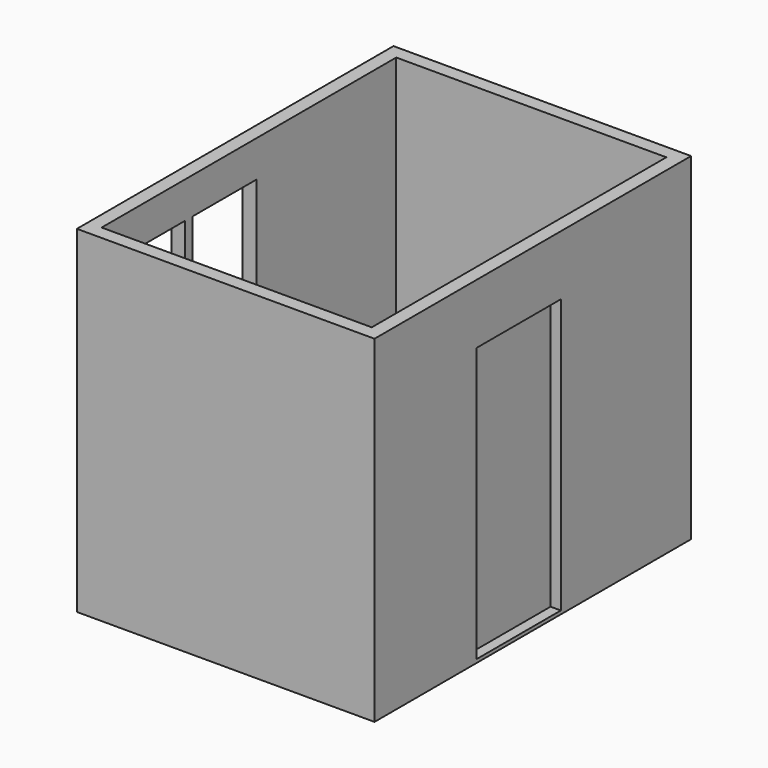
from build123d import *

# Parameters (mm, degrees)
F0_W     = 100
F0_H     = 580
F0_H_2   = 68
F0_H_3   = 765
F1_DEPTH = 2430
F2_W     = 580
F2_H     = 890
F3_DEPTH = 100.001
F4_W     = 765
F4_H     = 1994
F5_DEPTH = 100
F6_W     = 760
F6_H     = 1989
F7_DEPTH = 25
F8_DEPTH = 25


with BuildPart() as f1:
    # F0 (on Top) → F1 (new body)
    with BuildSketch(Plane.XY):
        Polygon((0, -2680), (-1966, -2680), (-1966, -2500), (-2066, -2500), (-2066, -2780), (100, -2780), (100, -1850), (0, -1850), align=None)
        with Locations((-2016, -2210)):
            Rectangle(F0_W, F0_H)
        with Locations((-2016, -1886)):
            Rectangle(F0_W, F0_H_2)
        with Locations((-2016, -1562)):
            Rectangle(F0_W, F0_H)
        with Locations((50, -1467.5)):
            Rectangle(F0_W, F0_H_3)
        Polygon((0, 0), (0, -1085), (100, -1085), (100, 100), (-2066, 100), (-2066, -1272), (-1966, -1272), (-1966, 0), align=None)
    extrude(amount=F1_DEPTH)

    # F2 (on face) → F3 (cut, through all)
    with BuildSketch(Plane.YZ.offset(-1966)):
        with Locations((-1562, 1720)):
            Rectangle(F2_W, F2_H)
        with Locations((-2210, 1720)):
            Rectangle(F2_W, F2_H)
    extrude(amount=-F3_DEPTH, mode=Mode.SUBTRACT)

    # F4 (on face) → F5 (cut, through all)
    with BuildSketch(Plane.YZ.offset(100)):
        with Locations((-1467.5, 997)):
            Rectangle(F4_W, F4_H)
    extrude(amount=-F5_DEPTH, mode=Mode.SUBTRACT)

    # F0 (on Top) → F8 (join)
    with BuildSketch(Plane.XY):
        Polygon((0, -2680), (-1966, -2680), (-1966, -2500), (-2066, -2500), (-2066, -2780), (100, -2780), (100, -1850), (0, -1850), align=None)
        with Locations((-2016, -2210)):
            Rectangle(F0_W, F0_H)
        with Locations((50, -1467.5)):
            Rectangle(F0_W, F0_H_3)
        with Locations((-2016, -1886)):
            Rectangle(F0_W, F0_H_2)
        Polygon((0, 0), (0, -1085), (100, -1085), (100, 100), (-2066, 100), (-2066, -1272), (-1966, -1272), (-1966, 0), align=None)
        with Locations((-2016, -1562)):
            Rectangle(F0_W, F0_H)
        Polygon((-1966, -2500), (-1966, -2680), (0, -2680), (0, -1850), (0, -1085), (0, 0), (-1966, 0), (-1966, -1272), (-1966, -1852), (-1966, -1920), align=None)
    extrude(amount=-F8_DEPTH)


with BuildPart() as f7:
    # F6 (on face) → F7 (new body)
    with BuildSketch(Plane(origin=(0, 0, 0), x_dir=(0, -1, 0), z_dir=(-1, 0, 0))):
        with Locations((1467.5, 994.5)):
            Rectangle(F6_W, F6_H)
    extrude(amount=-F7_DEPTH)


solid = Compound([f1.part, f7.part])
